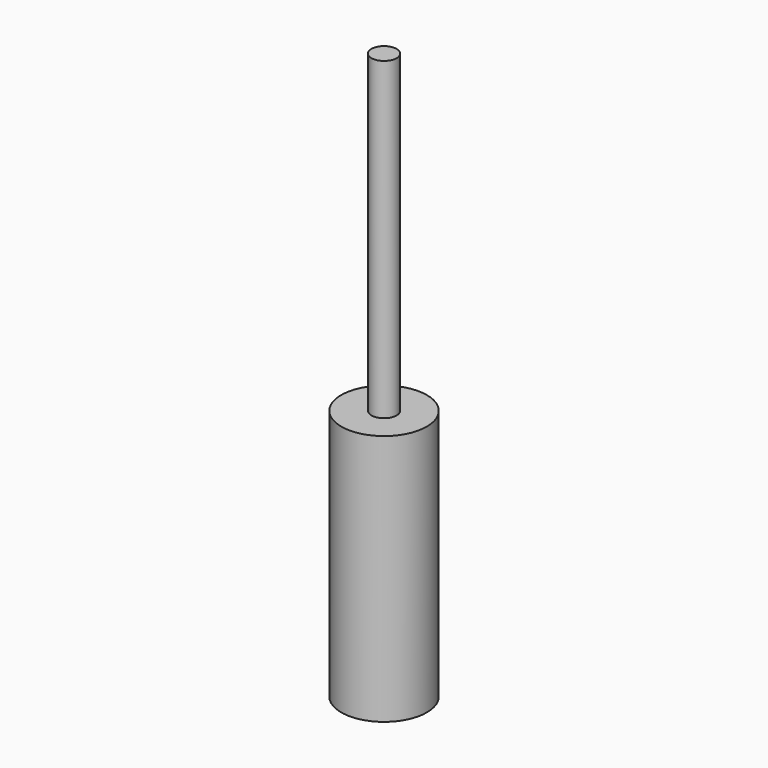
from build123d import *

# Parameters (mm, degrees)
F0_R     = 3.4
F0_R_2   = 1
F1_DEPTH = 20
F2_DEPTH = 25


# Not quite as in the source:
# - a feature names something its author has since deleted; it is built from what else it names


with BuildPart() as f1:
    # F0 (on Top) → F1 (new body)
    with BuildSketch(Plane.XY):
        Circle(F0_R)
        Circle(F0_R_2, mode=Mode.SUBTRACT)
        Circle(F0_R_2)
    extrude(amount=-F1_DEPTH)

    # F0 (on Top) → F2 (join)
    with BuildSketch(Plane.XY):
        Circle(F0_R_2)
    extrude(amount=F2_DEPTH)


solid = f1.part
